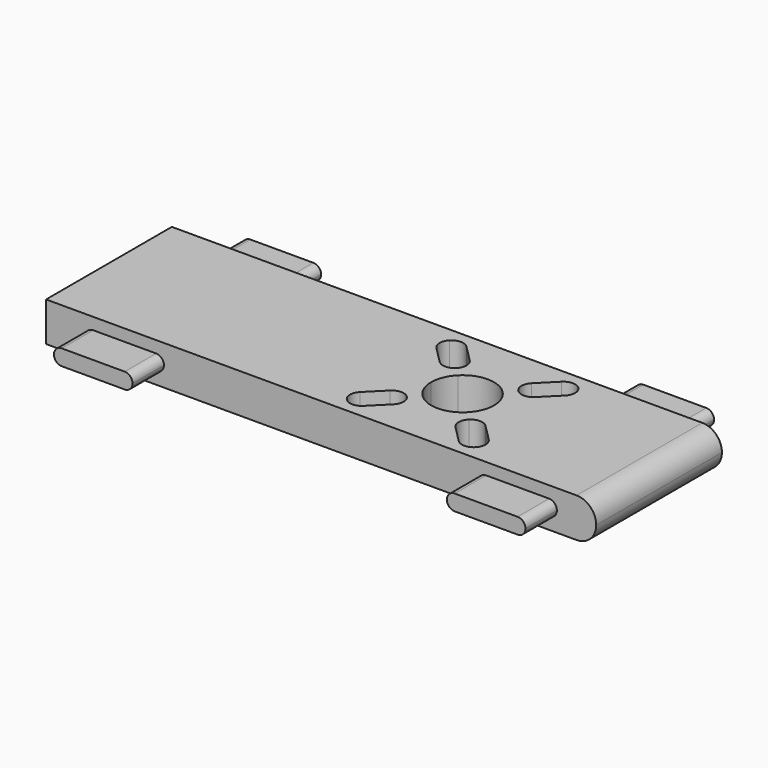
from build123d import *

# Parameters (mm, degrees)
F0_W     = 70
F0_H     = 20
F1_DEPTH = 5
F2_W     = 10
F2_H     = 2
F3_DEPTH = 5
F4_W     = 10
F4_H     = 2
F5_DEPTH = 5
F6_R     = 0.99999
F7_R     = 2.49999
F9_DEPTH = 5


# Not quite as in the source:
# - a fillet or chamfer is up to 0.001 mm smaller than in the source, because OpenCascade refuses the exact size


with BuildPart() as f1:
    # F0 (on Top) → F1 (new body)
    with BuildSketch(Plane.XY):
        Rectangle(F0_W, F0_H)
    extrude(amount=F1_DEPTH)

    # F2 (on face) → F3 (join)
    with BuildSketch(Plane.XZ.offset(10)):
        with Locations((-25, 2.5)):
            Rectangle(F2_W, F2_H)
        with Locations((25, 2.5)):
            Rectangle(F2_W, F2_H)
    extrude(amount=F3_DEPTH)

    # F4 (on face) → F5 (join)
    with BuildSketch(Plane(origin=(0, 10, 0), x_dir=(-1, 0, 0), z_dir=(0, 1, 0))):
        with Locations((-25, 2.5)):
            Rectangle(F4_W, F4_H)
        with Locations((25, 2.5)):
            Rectangle(F4_W, F4_H)
    extrude(amount=F5_DEPTH)

    # F6 (radius 1 in the source; OpenCascade refuses exactly that, so slightly less here)
    f6_edges = [f1.edges().sort_by_distance(p)[0] for p in [
        (30, 12.5, 3.5),
        (30, 12.5, 1.5),
        (20, 12.5, 3.5),
        (30, -12.5, 3.5),
        (30, -12.5, 1.5),
        (20, -12.5, 3.5),
        (-20, 12.5, 3.5),
        (-20, 12.5, 1.5),
        (-30, -12.5, 3.5),
        (-20, -12.5, 3.5),
        (-20, -12.5, 1.5),
        (-30, 12.5, 3.5),
        (20, 12.5, 1.5),
        (-30, 12.5, 1.5),
        (-30, -12.5, 1.5),
        (20, -12.5, 1.5),
    ]]
    fillet(f6_edges, radius=F6_R)

    # F7 (radius 2.5 in the source; OpenCascade refuses exactly that, so slightly less here)
    f7_edges = [f1.edges().sort_by_distance(p)[0] for p in [
        (35, 0, 5),
        (35, 0, 0),
    ]]
    fillet(f7_edges, radius=F7_R)

    # F8 (on face) → F9 (cut)
    with BuildSketch(Plane.XY.offset(5)):
        with BuildLine():
            Line((6.0606601718, -3.9393398282), (1.8180194847, -8.1819805153))
            ThreePointArc((1.8180194847, -8.1819805153), (2.8786796564, -8.6213203436), (3.9393398282, -8.1819805153))
            Line((3.9393398282, -8.1819805153), (6.0606601718, -6.0606601718))
            ThreePointArc((6.0606601718, -6.0606601718), (6.5, -5), (6.0606601718, -3.9393398282))
        make_face()
        with BuildLine():
            ThreePointArc((1.8180194847, -6.0606601718), (1.3786796564, -7.1213203436), (1.8180194847, -8.1819805153))
            Line((1.8180194847, -8.1819805153), (6.0606601718, -3.9393398282))
            ThreePointArc((6.0606601718, -3.9393398282), (5, -3.5), (3.9393398282, -3.9393398282))
            Line((3.9393398282, -3.9393398282), (1.8180194847, -6.0606601718))
        make_face()
        with BuildLine():
            ThreePointArc((7.1715728753, 2.8284271247), (6.30448187, 1.5307337295), (6, 0))
            Line((6, 0), (10, 0))
            Line((10, 0), (7.1715728753, 2.8284271247))
        make_face()
        with BuildLine():
            Line((10, 0), (6, 0))
            ThreePointArc((6, 0), (6.30448187, -1.5307337295), (7.1715728753, -2.8284271247))
            Line((7.1715728753, -2.8284271247), (10, 0))
        make_face()
        with BuildLine():
            Line((12.8284271247, -2.8284271247), (10, 0))
            Line((10, 0), (7.1715728753, -2.8284271247))
            ThreePointArc((7.1715728753, -2.8284271247), (10, -4), (12.8284271247, -2.8284271247))
        make_face()
        with BuildLine():
            Line((13.9393398282, -3.9393398282), (18.1819805153, -8.1819805153))
            ThreePointArc((18.1819805153, -8.1819805153), (18.6213203436, -7.1213203436), (18.1819805153, -6.0606601718))
            Line((18.1819805153, -6.0606601718), (16.0606601718, -3.9393398282))
            ThreePointArc((16.0606601718, -3.9393398282), (15, -3.5), (13.9393398282, -3.9393398282))
        make_face()
        with BuildLine():
            ThreePointArc((16.0606601718, -8.1819805153), (17.1213203436, -8.6213203436), (18.1819805153, -8.1819805153))
            Line((18.1819805153, -8.1819805153), (13.9393398282, -3.9393398282))
            ThreePointArc((13.9393398282, -3.9393398282), (13.5, -5), (13.9393398282, -6.0606601718))
            Line((13.9393398282, -6.0606601718), (16.0606601718, -8.1819805153))
        make_face()
        with BuildLine():
            ThreePointArc((18.1819805153, 6.0606601718), (18.6213203436, 7.1213203436), (18.1819805153, 8.1819805153))
            ThreePointArc((18.1819805153, 8.1819805153), (17.1213203436, 8.6213203436), (16.0606601718, 8.1819805153))
            Line((16.0606601718, 8.1819805153), (13.9393398282, 6.0606601718))
            ThreePointArc((13.9393398282, 6.0606601718), (13.5, 5), (13.9393398282, 3.9393398282))
            ThreePointArc((13.9393398282, 3.9393398282), (15, 3.5), (16.0606601718, 3.9393398282))
            Line((16.0606601718, 3.9393398282), (18.1819805153, 6.0606601718))
        make_face()
        with BuildLine():
            ThreePointArc((3.9393398282, 8.1819805153), (2.8786796564, 8.6213203436), (1.8180194847, 8.1819805153))
            ThreePointArc((1.8180194847, 8.1819805153), (1.3786796564, 7.1213203436), (1.8180194847, 6.0606601718))
            Line((1.8180194847, 6.0606601718), (3.9393398282, 3.9393398282))
            ThreePointArc((3.9393398282, 3.9393398282), (5, 3.5), (6.0606601718, 3.9393398282))
            ThreePointArc((6.0606601718, 3.9393398282), (6.5, 5), (6.0606601718, 6.0606601718))
            Line((6.0606601718, 6.0606601718), (3.9393398282, 8.1819805153))
        make_face()
        with BuildLine():
            Line((7.1715728753, 2.8284271247), (10, 0))
            Line((10, 0), (12.8284271247, 2.8284271247))
            ThreePointArc((12.8284271247, 2.8284271247), (10, 4), (7.1715728753, 2.8284271247))
        make_face()
        with BuildLine():
            Line((12.8284271247, 2.8284271247), (10, 0))
            Line((10, 0), (14, 0))
            ThreePointArc((14, 0), (13.69551813, 1.5307337295), (12.8284271247, 2.8284271247))
        make_face()
        with BuildLine():
            Line((14, 0), (10, 0))
            Line((10, 0), (12.8284271247, -2.8284271247))
            ThreePointArc((12.8284271247, -2.8284271247), (13.69551813, -1.5307337295), (14, 0))
        make_face()
    extrude(amount=-F9_DEPTH, mode=Mode.SUBTRACT)


solid = f1.part
